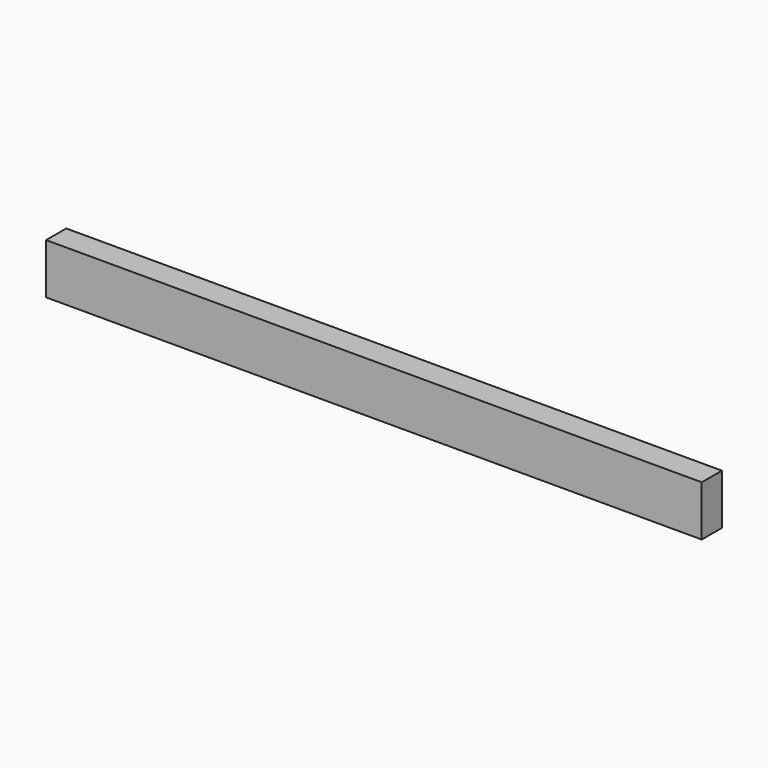
from build123d import *

# Parameters (mm, degrees)
F0_W     = 330.2
F0_H     = 25.4
F1_DEPTH = 12.7


# Not quite as in the source:
# - a feature names something its author has since deleted; it is built from what else it names


with BuildPart() as f1:
    # F0 (on Front) → F1 (new body)
    with BuildSketch(Plane.XZ):
        Rectangle(F0_W, F0_H)
    extrude(amount=F1_DEPTH)


solid = f1.part
